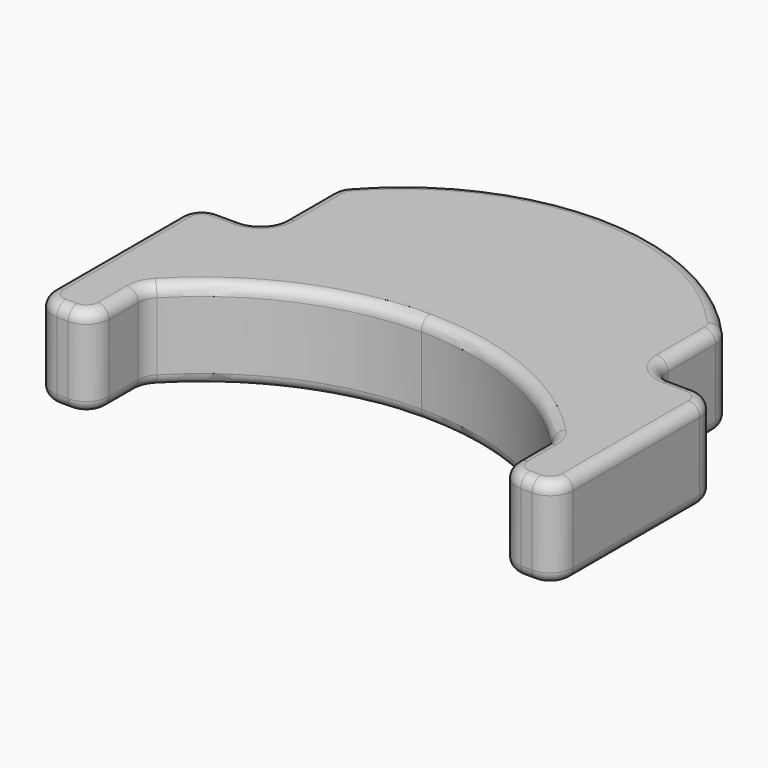
from build123d import *

# Parameters (mm, degrees)
F1_DEPTH = 4
F2_R     = 1
F3_R     = 0.5


# Not quite as in the source:
# - a feature names something its author has since deleted; it is built from what else it names


with BuildPart() as f1:
    # F0 (on Top) → F1 (new body)
    with BuildSketch(Plane.XY):
        with BuildLine():
            Line((9, -10), (9, -13))
            Line((9, -13), (11.5, -13))
            Line((11.5, -13), (11.5, -4))
            Line((11.5, -4), (8.5, -4))
            Line((8.5, -4), (8.5, 0))
            ThreePointArc((8.5, 0), (4.697073557, 2.9500313087), (0, 4))
            ThreePointArc((0, 4), (-4.697073557, 2.9500313087), (-8.5, 0))
            Line((-8.5, 0), (-8.5, -4))
            Line((-8.5, -4), (-11.5, -4))
            Line((-11.5, -4), (-11.5, -13))
            Line((-11.5, -13), (-9, -13))
            Line((-9, -13), (-9, -10))
            ThreePointArc((-9, -10), (-4.9244289009, -7.045034973), (0, -6))
            ThreePointArc((0, -6), (4.9244289009, -7.045034973), (9, -10))
        make_face()
    extrude(amount=F1_DEPTH)

    # F2
    f2_edges = [f1.edges().sort_by_distance(p)[0] for p in [
        (-9, -13, 2),
        (9, -13, 2),
        (-11.5, -4, 2),
        (-8.5, -4, 2),
        (8.5, -4, 2),
        (11.5, -4, 2),
        (9, -10, 2),
        (-9, -10, 2),
        (-11.5, -13, 2),
        (-8.5, 0, 2),
        (8.5, 0, 2),
        (11.5, -13, 2),
    ]]
    fillet(f2_edges, radius=F2_R)

    # F3
    f3_edges = [f1.edges().sort_by_distance(p)[0] for p in [
        (-9, -11.197088, 4),
        (0, -6, 4),
        (8.927119, -10.019411, 4),
        (-8.927119, -10.019411, 4),
        (9, -11.197088, 4),
        (9.292893, -12.707107, 4),
        (-9.292893, -12.707107, 4),
        (10.25, -13, 4),
        (-10.25, -13, 4),
        (11.207107, -12.707107, 4),
        (-11.207107, -12.707107, 4),
        (11.5, -8.5, 4),
        (-11.5, -8.5, 4),
        (11.207107, -4.292893, 4),
        (-11.207107, -4.292893, 4),
        (10, -4, 4),
        (-10, -4, 4),
        (8.792893, -3.707107, 4),
        (-8.792893, -3.707107, 4),
        (8.5, -1.68486, 4),
        (-8.5, -1.68486, 4),
        (8.43479, -0.014519, 4),
        (-8.43479, -0.014519, 4),
        (0, 4, 4),
        (10.25, -13, 0),
        (9, -11.197088, 0),
        (-9, -11.197088, 0),
        (-10.25, -13, 0),
        (0, -6, 0),
        (8.927119, -10.019411, 0),
        (9.292893, -12.707107, 0),
        (-8.927119, -10.019411, 0),
        (11.207107, -12.707107, 0),
        (11.5, -8.5, 0),
        (-9.292893, -12.707107, 0),
        (11.207107, -4.292893, 0),
        (10, -4, 0),
        (-11.207107, -12.707107, 0),
        (8.792893, -3.707107, 0),
        (-11.5, -8.5, 0),
        (8.5, -1.68486, 0),
        (-11.207107, -4.292893, 0),
        (8.43479, -0.014519, 0),
        (-10, -4, 0),
        (0, 4, 0),
        (-8.792893, -3.707107, 0),
        (-8.43479, -0.014519, 0),
        (-8.5, -1.68486, 0),
    ]]
    fillet(f3_edges, radius=F3_R)


solid = f1.part
